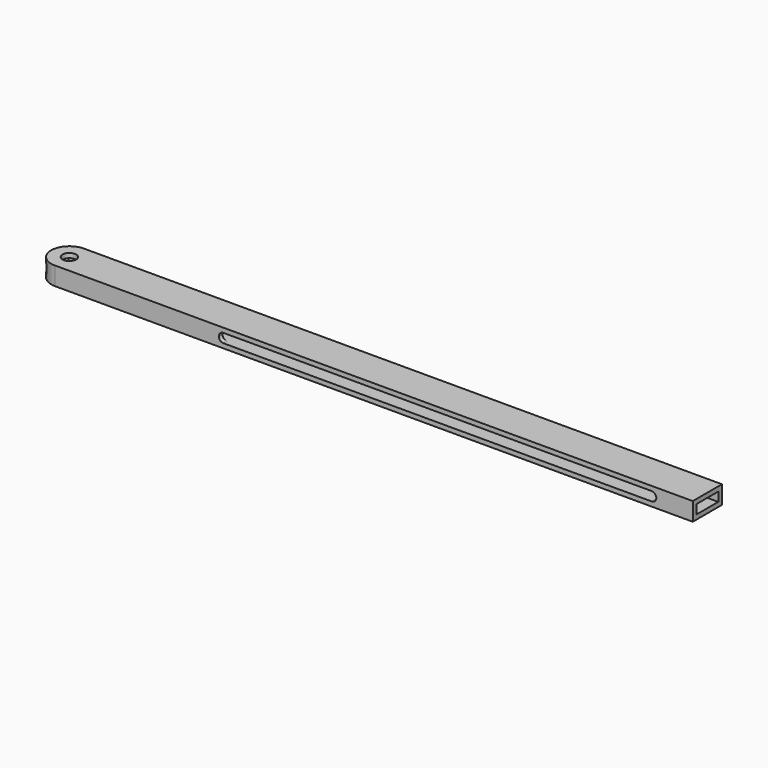
from build123d import *

# Parameters (mm, degrees)
F0_W          = 457.2
F0_H          = 25.4
F1_DEPTH      = 6.35
F2_R          = 12.69999
F3_R          = 4.7625
F4_DEPTH      = 12.701
F5_W          = 19.05
F5_H          = 6.35
F6_DEPTH      = 228.601
F6_DEPTH_BACK = 228.601
F7_W          = 304.8
F7_H          = 6.35
F8_DEPTH      = 12.701
F9_R          = 3.17499


# Not quite as in the source:
# - a fillet or chamfer is up to 0.001 mm smaller than in the source, because OpenCascade refuses the exact size


with BuildPart() as f1:
    # F0 (on Top) → F1 (new body, symmetric)
    with BuildSketch(Plane.XY):
        Rectangle(F0_W, F0_H)
    extrude(amount=F1_DEPTH, both=True)

    # F2 (radius 12.7 in the source; OpenCascade refuses exactly that, so slightly less here)
    f2_edges = [f1.edges().sort_by_distance(p)[0] for p in [
        (-228.6, 12.7, 0),
        (-228.6, -12.7, 0),
    ]]
    fillet(f2_edges, radius=F2_R)

    # F3 (on face) → F4 (cut, through all)
    with BuildSketch(Plane(origin=(0, 0, -6.35), x_dir=(1, 0, 0), z_dir=(0, 0, -1))):
        with Locations((-215.9, 0)):
            Circle(F3_R)
    extrude(amount=-F4_DEPTH, mode=Mode.SUBTRACT)

    # F5 (on Right) → F6 (cut, two sides)
    with BuildSketch(Plane.YZ) as f6_sk:
        Rectangle(F5_W, F5_H)
    extrude(amount=-F6_DEPTH, mode=Mode.SUBTRACT)
    extrude(f6_sk.sketch, amount=F6_DEPTH_BACK, mode=Mode.SUBTRACT)

    # F7 (on Front) → F8 (cut, through all)
    with BuildSketch(Plane.XZ):
        with Locations((50.8, 0)):
            Rectangle(F7_W, F7_H)
    extrude(amount=F8_DEPTH, mode=Mode.SUBTRACT)

    # F9 (radius 3.175 in the source; OpenCascade refuses exactly that, so slightly less here)
    f9_edges = [f1.edges().sort_by_distance(p)[0] for p in [
        (-101.6, -11.1125, 3.175),
        (203.2, -11.1125, -3.175),
        (203.2, -11.1125, 3.175),
        (-101.6, -11.1125, -3.175),
    ]]
    fillet(f9_edges, radius=F9_R)


solid = f1.part
